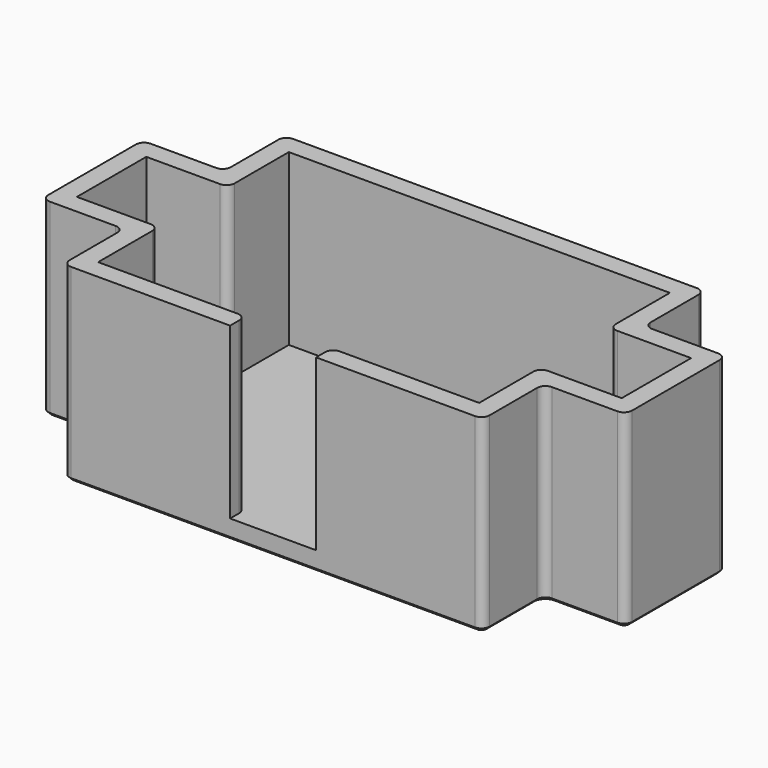
from build123d import *

# Parameters (mm, degrees)
F4_W      = 5.05
F4_H      = 5.35
F9_R      = 3
F10_DEPTH = 11.671
F11_R     = 0.5
F12_SIZE  = 0.2


with BuildPart() as f6:
    # F6: sweep along a path in F1
    with BuildLine(Plane.XZ) as f6_path:
        Line((0, 0), (0, 1.2))
        Line((0, 1.2), (0, 3.4))
        Line((0, 3.4), (0, 4.67))
        Line((0, 4.67), (0, 11.67))
    # F5 (on Top) → F6 (sweep)
    with BuildSketch(Plane.XY):
        Polygon((-12.95, -8.55), (0, -8.55), (12.95, -8.55), (12.95, -3.875), (18, -3.875), (18, 3.875), (12.95, 3.875), (12.95, 8.55), (-12.95, 8.55), (-12.95, 3.875), (-18, 3.875), (-18, -3.875), (-12.95, -3.875), align=None)
    sweep(path=f6_path.line)

    # F7: sweep along a path in F1
    with BuildLine(Plane.XZ) as f7_path:
        Line((0, 1.2), (0, 3.4))
        Line((0, 3.4), (0, 4.67))
        Line((0, 4.67), (0, 11.67))
    # F4 (on line) → F7 (sweep, cut)
    with BuildSketch(Plane.XY.offset(1.2)):
        Polygon((11.75, 2.675), (11.75, 7.35), (-11.75, 7.35), (-11.75, 2.675), (-11.75, -2.675), (-11.75, -7.35), (-2.65, -7.35), (-2.65, -16.2557040095), (2.65, -16.2557040095), (2.65, -7.35), (11.75, -7.35), (11.75, -2.675), align=None)
        with Locations((14.275, 0)):
            Rectangle(F4_W, F4_H)
        with Locations((-14.275, 0)):
            Rectangle(F4_W, F4_H)
    sweep(path=f7_path.line, mode=Mode.SUBTRACT)

    # F8: sweep along a path in F1
    with BuildLine(Plane.XZ) as f8_path:
        Line((0, 1.2), (0, 3.4))
    # F4 (on line) → F8 (sweep)
    with BuildSketch(Plane.XY.offset(1.2)):
        with Locations((-14.275, 0)):
            Rectangle(F4_W, F4_H)
        with Locations((14.275, 0)):
            Rectangle(F4_W, F4_H)
    sweep(path=f8_path.line)

    # F9 (on Top) → F10 (cut, through all)
    with BuildSketch(Plane.XY):
        Circle(F9_R)
    extrude(amount=F10_DEPTH, mode=Mode.SUBTRACT)

    # F11
    f11_edges = [f6.edges().sort_by_distance(p)[0] for p in [
        (-2.65, -7.35, 6.435),
        (2.65, -7.35, 6.435),
        (-11.75, 0, 3.4),
        (11.75, 0, 3.4),
        (18, -3.875, 5.835),
        (18, 3.875, 5.835),
        (12.95, -8.55, 5.835),
        (12.95, 8.55, 5.835),
        (-12.95, -8.55, 5.835),
        (-18, -3.875, 5.835),
        (-12.95, 8.55, 5.835),
        (-18, 3.875, 5.835),
        (12.95, 3.875, 5.835),
        (12.95, -3.875, 5.835),
        (-12.95, -3.875, 5.835),
        (-12.95, 3.875, 5.835),
        (11.75, 2.675, 7.535),
        (11.75, -2.675, 7.535),
        (-11.75, -2.675, 7.535),
        (-11.75, 2.675, 7.535),
    ]]
    fillet(f11_edges, radius=F11_R)

    # F12
    f12_edges = [f6.edges().sort_by_distance(p)[0] for p in [
        (0, -8.55, 0),
        (-12.803553, -8.403553, 0),
        (12.803553, -8.403553, 0),
        (-12.95, -6.2125, 0),
        (12.95, -6.2125, 0),
        (-13.096447, -4.021447, 0),
        (13.096447, -4.021447, 0),
        (-15.475, -3.875, 0),
        (15.475, -3.875, 0),
        (-17.853553, -3.728553, 0),
        (17.853553, -3.728553, 0),
        (-18, 0, 0),
        (18, 0, 0),
        (-17.853553, 3.728553, 0),
        (17.853553, 3.728553, 0),
        (-15.475, 3.875, 0),
        (15.475, 3.875, 0),
        (-13.096447, 4.021447, 0),
        (13.096447, 4.021447, 0),
        (-12.95, 6.2125, 0),
        (12.95, 6.2125, 0),
        (-12.803553, 8.403553, 0),
        (12.803553, 8.403553, 0),
        (0, 8.55, 0),
        (-3, 0, 0),
    ]]
    chamfer(f12_edges, length=F12_SIZE)


solid = f6.part
